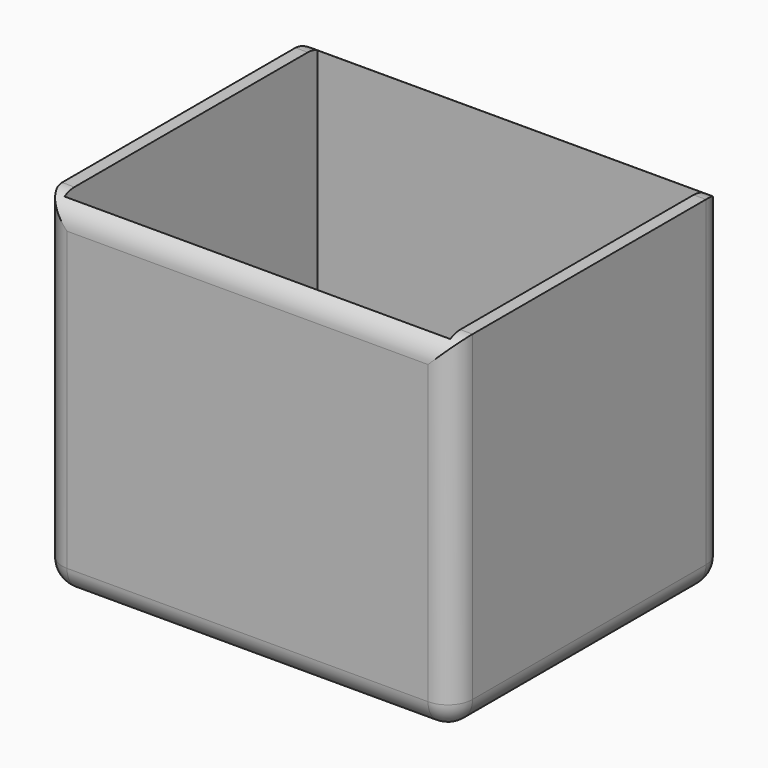
from build123d import *

# Parameters (mm, degrees)
F0_W         = 84.3196734786
F0_H         = 70.0790211558
F1_DEPTH     = 71.12
F2_T         = -2.54
F3_T1_DEPTH  = 78.74
F3_T3_DEPTH  = 109.7196734786
F3_T5_DEPTH  = 74.1596734786
F3_T7_DEPTH  = 59.9190211558
F3_S11_W     = 5.08
F3_S11_H     = 5.08
F3_T12_DEPTH = 5.08
F3_S17_W     = 5.08
F3_S17_H     = 5.08
F3_T18_DEPTH = 5.08
F3_S23_W     = 5.08
F3_S23_H     = 5.08
F3_T24_DEPTH = 5.08
F3_S29_W     = 5.08
F3_S29_H     = 5.08
F3_T30_DEPTH = 5.08


# Not quite as in the source:
# - a fillet or chamfer that OpenCascade refuses, or shapes differently, is made with other operations: its cross-section is extruded or revolved along the edge and cut away or added


with BuildPart() as f1:
    # F0 (on Top) → F1 (new body)
    with BuildSketch(Plane.XY):
        with Locations((-0.5621314049, -4.3096728623)):
            Rectangle(F0_W, F0_H)
    extrude(amount=F1_DEPTH)

    # F2
    f2_openings = [f1.faces().sort_by_distance(p)[0] for p in [
        (-0.562131, -4.309673, 71.12),
    ]]
    offset(amount=F2_T, openings=f2_openings)

    # F3: fillet of radius 5.08 on 10 edges, made by hand

    # F3_s2 → F3_t1 (cut)
    with BuildSketch(Plane.XY.offset(5.08)):
        with BuildLine():
            ThreePointArc((36.5177053344, -39.3491834402), (40.1098077829, -37.8612858886), (41.5977053344, -34.2691834402))
            Line((41.5977053344, -34.2691834402), (41.5977053344, -39.3491834402))
            Line((41.5977053344, -39.3491834402), (36.5177053344, -39.3491834402))
        make_face()
        with BuildLine():
            ThreePointArc((-42.7219681442, -34.2691834402), (-41.2340705926, -37.8612858886), (-37.6419681442, -39.3491834402))
            Line((-37.6419681442, -39.3491834402), (-42.7219681442, -39.3491834402))
            Line((-42.7219681442, -39.3491834402), (-42.7219681442, -34.2691834402))
        make_face()
        with BuildLine():
            ThreePointArc((36.5177053344, 30.7298377156), (40.1098077829, 29.2419401641), (41.5977053344, 25.6498377156))
            Line((41.5977053344, 25.6498377156), (41.5977053344, 30.7298377156))
            Line((41.5977053344, 30.7298377156), (36.5177053344, 30.7298377156))
        make_face()
        with BuildLine():
            ThreePointArc((-37.6419681442, 30.7298377156), (-41.2340705926, 29.2419401641), (-42.7219681442, 25.6498377156))
            Line((-42.7219681442, 25.6498377156), (-42.7219681442, 30.7298377156))
            Line((-42.7219681442, 30.7298377156), (-37.6419681442, 30.7298377156))
        make_face()
    extrude(amount=F3_T1_DEPTH, mode=Mode.SUBTRACT)

    # F3_s4 → F3_t3 (cut)
    with BuildSketch(Plane.YZ.offset(-55.4219681442)):
        with BuildLine():
            ThreePointArc((30.7298377156, 66.04), (29.2419401641, 69.6321024484), (25.6498377156, 71.12))
            Line((25.6498377156, 71.12), (30.7298377156, 71.12))
            Line((30.7298377156, 71.12), (30.7298377156, 66.04))
        make_face()
        with BuildLine():
            ThreePointArc((-39.3491834402, 66.04), (-37.8612858886, 69.6321024484), (-34.2691834402, 71.12))
            Line((-34.2691834402, 71.12), (-39.3491834402, 71.12))
            Line((-39.3491834402, 71.12), (-39.3491834402, 66.04))
        make_face()
    extrude(amount=F3_T3_DEPTH, mode=Mode.SUBTRACT)

    # F3_s6 → F3_t5 (cut)
    with BuildSketch(Plane.YZ.offset(-37.6419681442)):
        with BuildLine():
            ThreePointArc((30.7298377156, 5.08), (29.2419401641, 1.4878975516), (25.6498377156, 0))
            Line((25.6498377156, 0), (30.7298377156, 0))
            Line((30.7298377156, 0), (30.7298377156, 5.08))
        make_face()
        with BuildLine():
            ThreePointArc((-39.3491834402, 5.08), (-37.8612858886, 1.4878975516), (-34.2691834402, 0))
            Line((-34.2691834402, 0), (-39.3491834402, 0))
            Line((-39.3491834402, 0), (-39.3491834402, 5.08))
        make_face()
    extrude(amount=F3_T5_DEPTH, mode=Mode.SUBTRACT)

    # F3_s8 → F3_t7 (cut)
    with BuildSketch(Plane.XZ.offset(-25.6498377156)):
        with BuildLine():
            ThreePointArc((41.5977053344, 5.08), (40.1098077829, 1.4878975516), (36.5177053344, 0))
            Line((36.5177053344, 0), (41.5977053344, 0))
            Line((41.5977053344, 0), (41.5977053344, 5.08))
        make_face()
        with BuildLine():
            ThreePointArc((-42.7219681442, 5.08), (-41.2340705926, 1.4878975516), (-37.6419681442, 0))
            Line((-37.6419681442, 0), (-42.7219681442, 0))
            Line((-42.7219681442, 0), (-42.7219681442, 5.08))
        make_face()
    extrude(amount=F3_T7_DEPTH, mode=Mode.SUBTRACT)


with BuildPart() as f3_tool10:
    # F3_s11 → F3_t12 (new body)
    with BuildSketch(Plane.XZ.offset(34.2691834402)):
        with Locations((39.0577053344, 2.54)):
            Rectangle(F3_S11_W, F3_S11_H)
    extrude(amount=F3_T12_DEPTH)

    # F3_s13 → F3_t14 (revolve, cut)
    with BuildSketch(Plane(origin=(36.5177053344, -34.2691834402, 5.08), x_dir=(-0.7071067812, 0, 0.7071067812), z_dir=(0.7071067812, 0, 0.7071067812))):
        with BuildLine():
            ThreePointArc((0, -5.08), (5.08, 0), (0, 5.08))
            Line((0, 5.08), (0, -5.08))
        make_face()
    revolve(axis=Axis((36.5177053344, -34.2691834402, 5.08), (0, -1, 0)), mode=Mode.SUBTRACT)


with BuildPart() as f1_1:
    add(f1.part)

    # F3_t9: cut F3_tool10
    add(f3_tool10.part, mode=Mode.SUBTRACT)


with BuildPart() as f3_tool16:
    # F3_s17 → F3_t18 (new body)
    with BuildSketch(Plane.YZ.offset(-37.6419681442)):
        with Locations((-36.8091834402, 2.54)):
            Rectangle(F3_S17_W, F3_S17_H)
    extrude(amount=-F3_T18_DEPTH)

    # F3_s19 → F3_t20 (revolve, cut)
    with BuildSketch(Plane(origin=(-37.6419681442, -34.2691834402, 5.08), x_dir=(0, 0.7071067812, 0.7071067812), z_dir=(0, -0.7071067812, 0.7071067812))):
        with BuildLine():
            ThreePointArc((0, -5.08), (5.08, 0), (0, 5.08))
            Line((0, 5.08), (0, -5.08))
        make_face()
    revolve(axis=Axis((-37.6419681442, -34.2691834402, 5.08), (-1, 0, 0)), mode=Mode.SUBTRACT)


with BuildPart() as f1_2:
    add(f1_1.part)

    # F3_t15: cut F3_tool16
    add(f3_tool16.part, mode=Mode.SUBTRACT)


with BuildPart() as f3_tool22:
    # F3_s23 → F3_t24 (new body)
    with BuildSketch(Plane.XZ.offset(-25.6498377156)):
        with Locations((39.0577053344, 2.54)):
            Rectangle(F3_S23_W, F3_S23_H)
    extrude(amount=-F3_T24_DEPTH)

    # F3_s25 → F3_t26 (revolve, cut)
    with BuildSketch(Plane(origin=(36.5177053344, 25.6498377156, 5.08), x_dir=(-0.7071067812, 0, 0.7071067812), z_dir=(-0.7071067812, 0, -0.7071067812))):
        with BuildLine():
            ThreePointArc((0, -5.08), (5.08, 0), (0, 5.08))
            Line((0, 5.08), (0, -5.08))
        make_face()
    revolve(axis=Axis((36.5177053344, 25.6498377156, 5.08), (0, 1, 0)), mode=Mode.SUBTRACT)


with BuildPart() as f1_3:
    add(f1_2.part)

    # F3_t21: cut F3_tool22
    add(f3_tool22.part, mode=Mode.SUBTRACT)


with BuildPart() as f3_tool28:
    # F3_s29 → F3_t30 (new body)
    with BuildSketch(Plane.XZ.offset(-25.6498377156)):
        with Locations((-40.1819681442, 2.54)):
            Rectangle(F3_S29_W, F3_S29_H)
    extrude(amount=-F3_T30_DEPTH)

    # F3_s31 → F3_t32 (revolve, cut)
    with BuildSketch(Plane(origin=(-37.6419681442, 25.6498377156, 5.08), x_dir=(0.7071067812, 0, 0.7071067812), z_dir=(-0.7071067812, 0, 0.7071067812))):
        with BuildLine():
            ThreePointArc((0, -5.08), (5.08, 0), (0, 5.08))
            Line((0, 5.08), (0, -5.08))
        make_face()
    revolve(axis=Axis((-37.6419681442, 25.6498377156, 5.08), (0, 1, 0)), mode=Mode.SUBTRACT)


with BuildPart() as f1_4:
    add(f1_3.part)

    # F3_t27: cut F3_tool28
    add(f3_tool28.part, mode=Mode.SUBTRACT)


solid = f1_4.part
